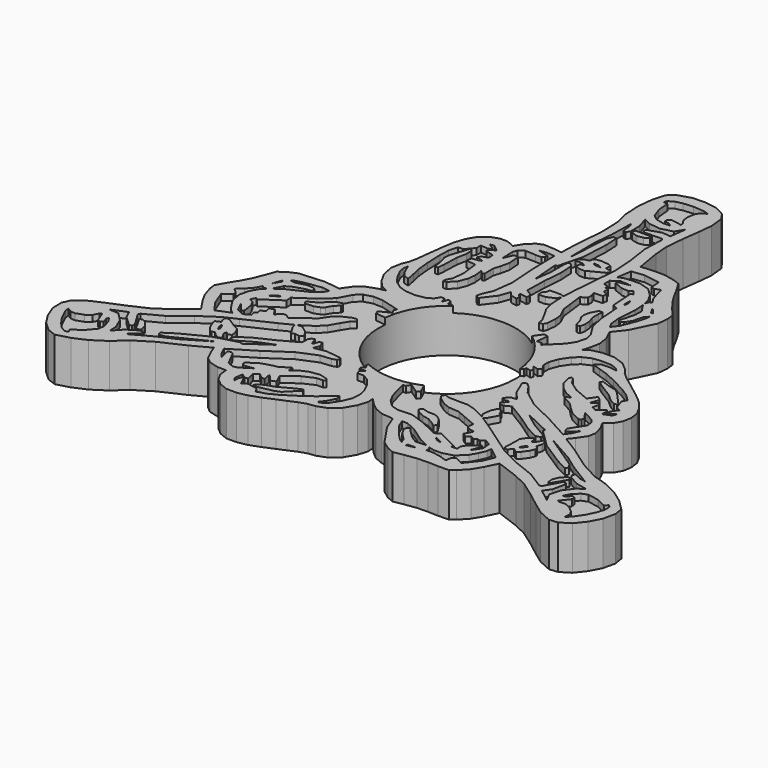
from build123d import *

# Parameters (mm, degrees)
F0_R            = 13.4
F0_R_2          = 11
F2_DEPTH        = 7
F3_DEPTH        = 7
F3_COPIES_COUNT = 3
F5_DEPTH        = 1
F5_COPIES_COUNT = 3
F6_R            = 0.2588079951
F6_R_2          = 0.2097461611
F6_R_3          = 0.2076285379
F7_DEPTH        = 7


# Not quite as in the source:
# - a pattern or mirror of a feature is missing from the dataset's text; its kind, count and spacing are read off the source's solid


with BuildPart() as f2:
    # F0 (on Top) → F2 (new body)
    with BuildSketch(Plane.XY):
        Circle(F0_R)
        Circle(F0_R_2, mode=Mode.SUBTRACT)
    extrude(amount=F2_DEPTH)

    # F1 (on Top) → F3 (join)
    with BuildSketch(Plane.XY):
        with BuildLine():
            ThreePointArc((-11.6641876562, 6.5959628805), (-0.1636582331, 13.3990005591), (11.4996029427, 6.8788903291))
            Line((11.4996029427, 6.8788903291), (12.5380335376, 7.9339332879))
            Line((12.5380335376, 7.9339332879), (13.6808827519, 9.3602091074))
            Line((13.6808827519, 9.3602091074), (14.2020219937, 11.0150557011))
            Line((14.2020219937, 11.0150557011), (14.4671630114, 12.5236166641))
            Line((14.4671630114, 12.5236166641), (14.256878756, 14.1144637018))
            Line((14.256878756, 14.1144637018), (13.4705984965, 15.7601684332))
            Line((13.4705984965, 15.7601684332), (14.9883022532, 17.6892988384))
            Line((14.9883022532, 17.6892988384), (16.7711470276, 21.3647019118))
            Line((16.7711470276, 21.3647019118), (16.9540029019, 23.0104047805))
            Line((16.9540029019, 23.0104047805), (16.8077182025, 24.2081098258))
            Line((16.8077182025, 24.2081098258), (15.7380122691, 25.497244671))
            Line((15.7380122691, 25.497244671), (14.6043049172, 26.941806078))
            Line((14.6043049172, 26.941806078), (13.6717399582, 28.4503661096))
            Line((13.6717399582, 28.4503661096), (12.9220308736, 29.8675000668))
            Line((12.9220308736, 29.8675000668), (12.0077515021, 31.3760600984))
            Line((12.0077515021, 31.3760600984), (11.1026149243, 31.741771847))
            Line((11.1026149243, 31.741771847), (9.3380557373, 32.1531966329))
            Line((9.3380557373, 32.1531966329), (7.6283533126, 32.1714803576))
            Line((7.6283533126, 32.1714803576), (5.4432251491, 32.0251956582))
            Line((5.4432251491, 32.0251956582), (4.7849440016, 35.9017364681))
            Line((4.7849440016, 35.9017364681), (4.6020881273, 38.2605791092))
            Line((4.6020881273, 38.2605791092), (4.8763719387, 41.2319898605))
            Line((4.8763719387, 41.2319898605), (5.2420832217, 44.0388247371))
            Line((5.2420832217, 44.0388247371), (5.4706535302, 46.2513826787))
            Line((5.4706535302, 46.2513826787), (5.242082756, 48.4639406204))
            Line((5.242082756, 48.4639406204), (4.4466597028, 49.5885051787))
            Line((4.4466597028, 49.5885051787), (2.8375282418, 50.4570677876))
            Line((2.8375282418, 50.4570677876), (0.8443988045, 50.7496409118))
            Line((0.8443988045, 50.7496409118), (-1.194444485, 50.6673529744))
            Line((-1.194444485, 50.6673529744), (-3.1052886043, 50.0639304519))
            Line((-3.1052886043, 50.0639304519), (-4.2572808452, 49.1222254932))
            Line((-4.2572808452, 49.1222254932), (-4.8241345212, 46.9736680388))
            Line((-4.8241345212, 46.9736680388), (-5.0709899515, 44.6788258851))
            Line((-5.0709899515, 44.6788258851), (-4.9338475801, 42.0639887452))
            Line((-4.9338475801, 42.0639887452), (-4.3761371635, 39.5588614047))
            Line((-4.3761371635, 39.5588614047), (-4.2755664326, 36.2948812544))
            Line((-4.2755664326, 36.2948812544), (-4.6504209749, 32.0617668331))
            Line((-4.6504209749, 32.0617668331), (-4.7601344995, 28.843505308))
            Line((-4.7601344995, 28.843505308), (-5.9669832699, 29.0355049074))
            Line((-5.9669832699, 29.0355049074), (-7.6675429009, 29.1452184319))
            Line((-7.6675429009, 29.1452184319), (-8.7372502312, 28.7429355085))
            Line((-8.7372502312, 28.7429355085), (-9.8709575832, 27.6092290878))
            Line((-9.8709575832, 27.6092290878), (-10.5749526992, 26.4389514923))
            Line((-10.5749526992, 26.4389514923), (-11.8823722005, 26.9875191152))
            Line((-11.8823722005, 26.9875191152), (-13.1257921457, 26.9875191152))
            Line((-13.1257921457, 26.9875191152), (-14.4240688533, 26.5212375671))
            Line((-14.4240688533, 26.5212375671), (-15.5669180676, 25.625243783))
            Line((-15.5669180676, 25.625243783), (-16.3989141583, 24.2081116885))
            Line((-16.3989141583, 24.2081116885), (-16.9291961938, 22.6721223444))
            Line((-16.9291961938, 22.6721223444), (-17.2400511801, 20.9167040884))
            Line((-17.2400511801, 20.9167040884), (-17.4686219543, 19.0150048584))
            Line((-17.4686219543, 19.0150048584), (-17.6514778286, 17.6253002137))
            Line((-17.6514778286, 17.6253002137), (-17.8069043905, 16.1898806691))
            Line((-17.8069043905, 16.1898806691), (-18.0811882019, 14.9098904803))
            Line((-18.0811882019, 14.9098904803), (-18.5291860253, 13.8401836157))
            Line((-18.5291860253, 13.8401836157), (-18.8020132482, 12.2613888234))
            Line((-18.8020132482, 12.2613888234), (-18.4454452246, 10.3779723868))
            Line((-18.4454452246, 10.3779723868), (-17.4945946783, 8.6956974119))
            Line((-17.4945946783, 8.6956974119), (-16.4157431573, 7.5345630758))
            Line((-16.4157431573, 7.5345630758), (-14.9711817503, 6.821425166))
            Line((-14.9711817503, 6.821425166), (-13.2554527372, 6.4937388524))
            Line((-13.2554527372, 6.4937388524), (-11.6641876562, 6.5959628805))
        make_face()
    f3 = extrude(amount=F3_DEPTH)

    # F3_copies: F3 ×3 about axis
    f3_copies_axis = Axis((0, 0, 0), (0, 0, 1))
    for i in range(1, F3_COPIES_COUNT):
        add(f3.rotate(f3_copies_axis, i * 360 / F3_COPIES_COUNT))

    # F4 (on face) → F5 (cut)
    with BuildSketch(Plane.XY.offset(7)):
        with BuildLine():
            Line((-6.7291953601, 9.3133719638), (-6.2807447637, 9.0306281738))
            ThreePointArc((-6.2807447637, 9.0306281738), (0.163569186, 10.9987838019), (6.5465070851, 8.8398667968))
            Line((6.5465070851, 8.8398667968), (7.4893734418, 10.1453736424))
            Line((7.4893734418, 10.1453736424), (8.0973692238, 10.0600402802))
            Line((8.0973692238, 10.0600402802), (7.9587036744, 8.1293871626))
            Line((7.9587036744, 8.1293871626), (8.7266983464, 8.1080542877))
            Line((8.7266983464, 8.1080542877), (8.9506972581, 7.692056708))
            Line((8.9506972581, 7.692056708), (11.1800152808, 9.9000418559))
            Line((11.1800152808, 9.9000418559), (11.9586763903, 11.1480327323))
            Line((11.9586763903, 11.1480327323), (12.3213399202, 12.5560229644))
            Line((12.3213399202, 12.5560229644), (12.0546752587, 13.7720145285))
            Line((12.0546752587, 13.7720145285), (10.8386827633, 15.6813338399))
            Line((10.8386827633, 15.6813338399), (10.3586865589, 18.0813185871))
            Line((10.3586865589, 18.0813185871), (10.1133547723, 21.3559605181))
            Line((10.1133547723, 21.3559605181), (9.2920269817, 21.7826254666))
            Line((9.2920269817, 21.7826254666), (9.0466951951, 25.4839323461))
            Line((9.0466951951, 25.4839323461), (9.4200260937, 25.601265952))
            Line((9.4200260937, 25.601265952), (8.8973622769, 26.3265930116))
            Line((8.8973622769, 26.3265930116), (8.3427000791, 25.9425956756))
            Line((8.3427000791, 25.9425956756), (7.2973738424, 25.9745959193))
            Line((7.2973738424, 25.9745959193), (5.6973844767, 26.6252588481))
            Line((5.6973844767, 26.6252588481), (5.8893831447, 26.9985888153))
            Line((5.8893831447, 26.9985888153), (7.7347038314, 27.2972546518))
            Line((7.7347038314, 27.2972546518), (5.8360504918, 27.414586395))
            Line((5.8360504918, 27.414586395), (4.7907242551, 26.646591723))
            Line((4.7907242551, 26.646591723), (4.7800578177, 25.5052670836))
            Line((4.7800578177, 25.5052670836), (5.4733860306, 25.3666006029))
            Line((5.4733860306, 25.3666006029), (5.5800522678, 24.8332712799))
            Line((5.5800522678, 24.8332712799), (6.0813818127, 24.6626045555))
            Line((6.0813818127, 24.6626045555), (6.0493825004, 23.8519441336))
            Line((6.0493825004, 23.8519441336), (6.7960438319, 23.6386116594))
            Line((6.7960438319, 23.6386116594), (6.7000444978, 22.8599514812))
            Line((6.7000444978, 22.8599514812), (5.2813878283, 22.774618119))
            Line((5.2813878283, 22.774618119), (5.5480524898, 22.0279563218))
            Line((5.5480524898, 22.0279563218), (5.5267191492, 21.3879607618))
            Line((5.5267191492, 21.3879607618), (5.1960549317, 21.0999622941))
            Line((5.1960549317, 21.0999622941), (4.6307253651, 20.8759643137))
            Line((4.6307253651, 20.8759643137), (4.9187233672, 18.5079798102))
            Line((4.9187233672, 18.5079798102), (5.0893891603, 17.0573238283))
            Line((5.0893891603, 17.0573238283), (5.8467173949, 15.4786678031))
            Line((5.8467173949, 15.4786678031), (5.9960498475, 14.3053419888))
            Line((5.9960498475, 14.3053419888), (5.8573838323, 12.7906855196))
            Line((5.8573838323, 12.7906855196), (5.5800522678, 12.2466897592))
            Line((5.5800522678, 12.2466897592), (4.9933898263, 12.1933566406))
            Line((4.9933898263, 12.1933566406), (4.8440573737, 13.0253508687))
            Line((4.8440573737, 13.0253508687), (4.2147282511, 14.2093431205))
            Line((4.2147282511, 14.2093431205), (3.3507344779, 15.7026667148))
            Line((3.3507344779, 15.7026667148), (2.9987369198, 17.0999895781))
            Line((2.9987369198, 17.0999895781), (2.8814044781, 19.3826407194))
            Line((2.8814044781, 19.3826407194), (2.550739795, 18.7426451594))
            Line((2.550739795, 18.7426451594), (1.228082343, 18.1773155928))
            Line((1.228082343, 18.1773155928), (0.1507562847, 18.1346479803))
            Line((0.1507562847, 18.1346479803), (0.022757129, 18.7639780343))
            Line((0.022757129, 18.7639780343), (0.4814206914, 19.339973107))
            Line((0.4814206914, 19.339973107), (0.5880866665, 19.8946371675))
            Line((0.5880866665, 19.8946371675), (2.4014078081, 19.9266355485))
            Line((2.4014078081, 19.9266355485), (2.9027375858, 19.7026375681))
            Line((2.9027375858, 19.7026375681), (3.0200700276, 21.8892898411))
            Line((3.0200700276, 21.8892898411), (3.4254004713, 26.8599223346))
            Line((3.4254004713, 26.8599223346), (3.6280651111, 29.2065739632))
            Line((3.6280651111, 29.2065739632), (3.3933999948, 32.5345508754))
            Line((3.3933999948, 32.5345508754), (2.8600706719, 36.1505262554))
            Line((2.8600706719, 36.1505262554), (2.9880695511, 39.3398366868))
            Line((2.9880695511, 39.3398366868), (2.7747380082, 39.6491698921))
            Line((2.7747380082, 39.6491698921), (-0.137241921, 39.5851694047))
            Line((-0.137241921, 39.5851694047), (-0.3612406144, 39.9158336222))
            Line((-0.3612406144, 39.9158336222), (-0.2652412222, 40.2784980834))
            Line((-0.2652412222, 40.2784980834), (1.8254109891, 40.9504920244))
            Line((1.8254109891, 40.9504920244), (3.1907348894, 40.8011600375))
            Line((3.1907348894, 40.8011600375), (3.5320662428, 43.4038117528))
            Line((3.5320662428, 43.4038117528), (2.7214051224, 42.1024858952))
            Line((2.7214051224, 42.1024858952), (0.8760846104, 41.6224896908))
            Line((0.8760846104, 41.6224896908), (-0.9799030377, 41.835822165))
            Line((-0.9799030377, 41.835822165), (-2.1425618324, 42.4331501126))
            Line((-2.1425618324, 42.4331501126), (-1.577232033, 40.6198278069))
            Line((-1.577232033, 40.6198278069), (-1.5345660504, 38.7745089829))
            Line((-1.5345660504, 38.7745089829), (-1.9078967161, 38.1878465414))
            Line((-1.9078967161, 38.1878465414), (-2.3665602785, 38.3265130222))
            Line((-2.3665602785, 38.3265130222), (-2.4732262827, 39.6385006607))
            Line((-2.4732262827, 39.6385006607), (-2.7505576145, 40.4064953327))
            Line((-2.7505576145, 40.4064953327), (-2.8572236188, 36.4278554916))
            Line((-2.8572236188, 36.4278554916), (-3.145221388, 33.5265398026))
            Line((-3.145221388, 33.5265398026), (-3.081221832, 28.523908928))
            Line((-3.081221832, 28.523908928), (-2.6438913774, 35.3505313396))
            Line((-2.6438913774, 35.3505313396), (-2.2385607008, 36.2038575113))
            Line((-2.2385607008, 36.2038575113), (-1.7265641363, 36.1611917615))
            Line((-1.7265641363, 36.1611917615), (-1.6198985977, 33.9212082326))
            Line((-1.6198985977, 33.9212082326), (-1.8332301406, 29.6119041741))
            Line((-1.8332301406, 29.6119041741), (-2.8358900454, 25.7079303265))
            Line((-2.8358900454, 25.7079303265), (-3.1772209331, 25.6439298391))
            Line((-3.1772209331, 25.6439298391), (-2.8145567048, 21.1319606751))
            Line((-2.8145567048, 21.1319606751), (-2.4412258063, 23.7559434026))
            Line((-2.4412258063, 23.7559434026), (-2.4305593688, 26.5719238669))
            Line((-2.4305593688, 26.5719238669), (-2.3132269271, 27.2119194269))
            Line((-2.3132269271, 27.2119194269), (-1.9718960393, 27.2439196706))
            Line((-1.9718960393, 27.2439196706), (-1.4598993585, 26.710588485))
            Line((-1.4598993585, 26.710588485), (-1.3319003629, 24.4706049562))
            Line((-1.3319003629, 24.4706049562), (-1.5772319166, 21.4946251363))
            Line((-1.5772319166, 21.4946251363), (-1.6518983757, 18.1559808552))
            Line((-1.6518983757, 18.1559808552), (-0.7239042316, 17.558651045))
            Line((-0.7239042316, 17.558651045), (-0.4785726778, 17.1213205904))
            Line((-0.4785726778, 17.1213205904), (-0.595905236, 16.6519898921))
            Line((-0.595905236, 16.6519898921), (-1.7798973713, 16.8759897351))
            Line((-1.7798973713, 16.8759897351), (-1.705231145, 16.545323655))
            Line((-1.705231145, 16.545323655), (-1.2359009124, 16.0759948194))
            Line((-1.2359009124, 16.0759948194), (-1.3425670331, 15.5853312463))
            Line((-1.3425670331, 15.5853312463), (-2.3452267051, 15.7773289829))
            Line((-2.3452267051, 15.7773289829), (-2.9425560497, 16.545323655))
            Line((-2.9425560497, 16.545323655), (-3.5612182692, 14.7853363305))
            Line((-3.5612182692, 14.7853363305), (-5.0865411758, 12.769350782))
            Line((-5.0865411758, 12.769350782), (-5.4385391995, 12.7586834133))
            Line((-5.4385391995, 12.7586834133), (-5.705203861, 13.0786811933))
            Line((-5.705203861, 13.0786811933), (-5.5345380679, 13.8466758654))
            Line((-5.5345380679, 13.8466758654), (-4.8305429518, 15.3933325782))
            Line((-4.8305429518, 15.3933325782), (-4.4252122752, 18.6146423221))
            Line((-4.4252122752, 18.6146423221), (-4.7345436178, 23.0092797428))
            Line((-4.7345436178, 23.0092797428), (-4.8412093893, 27.5532491505))
            Line((-4.8412093893, 27.5532491505), (-6.0038683005, 27.6599153876))
            Line((-6.0038683005, 27.6599153876), (-7.2198598646, 27.5319162756))
            Line((-7.2198598646, 27.5319162756), (-5.5238711648, 27.0412527025))
            Line((-5.5238711648, 27.0412527025), (-5.5558704771, 26.5612564981))
            Line((-5.5558704771, 26.5612564981), (-5.8972020634, 26.2839253992))
            Line((-5.8972020634, 26.2839253992), (-6.8678618409, 26.3159237802))
            Line((-6.8678618409, 26.3159237802), (-8.563850075, 26.4012571424))
            Line((-8.563850075, 26.4012571424), (-9.3638449907, 25.8145947009))
            Line((-9.3638449907, 25.8145947009), (-9.6198432148, 25.1319315284))
            Line((-9.6198432148, 25.1319315284), (-9.5451772213, 23.0199471116))
            Line((-9.5451772213, 23.0199471116), (-8.9265145361, 24.5132707059))
            Line((-8.9265145361, 24.5132707059), (-8.4678512067, 24.6199350804))
            Line((-8.4678512067, 24.6199350804), (-8.1691863015, 24.4066044688))
            Line((-8.1691863015, 24.4066044688), (-8.0411871895, 22.5719492882))
            Line((-8.0411871895, 22.5719492882), (-8.3611849695, 21.1212933064))
            Line((-8.3611849695, 21.1212933064), (-8.6811827496, 20.1399661601))
            Line((-8.6811827496, 20.1399661601), (-8.6598489434, 18.3479785919))
            Line((-8.6598489434, 18.3479785919), (-8.9585138485, 18.2093121111))
            Line((-8.9585138485, 18.2093121111), (-9.4598438591, 18.6999756843))
            Line((-9.4598438591, 18.6999756843), (-9.2998445034, 17.20665209))
            Line((-9.2998445034, 17.20665209), (-9.4385109842, 16.0226598382))
            Line((-9.4385109842, 16.0226598382), (-10.0038396195, 14.5720038563))
            Line((-10.0038396195, 14.5720038563), (-10.9745003283, 13.6226769537))
            Line((-10.9745003283, 13.6226769537), (-11.4651629701, 13.5480109602))
            Line((-11.4651629701, 13.5480109602), (-11.4758303389, 13.9640085399))
            Line((-11.4758303389, 13.9640085399), (-10.9638338909, 14.9026690051))
            Line((-10.9638338909, 14.9026690051), (-10.7825016603, 16.9079881161))
            Line((-10.7825016603, 16.9079881161), (-11.1238332465, 19.5426363498))
            Line((-11.1238332465, 19.5426363498), (-12.6598225906, 19.7026357055))
            Line((-12.6598225906, 19.7026357055), (-12.5104906037, 20.5346290022))
            Line((-12.5104906037, 20.5346290022), (-11.3691650331, 20.7159612328))
            Line((-11.3691650331, 20.7159612328), (-11.0278343782, 20.8759605885))
            Line((-11.0278343782, 20.8759605885), (-12.1798263863, 21.2706252933))
            Line((-12.1798263863, 21.2706252933), (-11.9238281623, 21.7292886227))
            Line((-11.9238281623, 21.7292886227), (-10.9318345785, 22.0492854714))
            Line((-10.9318345785, 22.0492854714), (-11.0278343782, 22.9239463806))
            Line((-11.0278343782, 22.9239463806), (-11.6891628131, 23.1052786112))
            Line((-11.6891628131, 23.1052786112), (-12.3718250543, 23.3399439603))
            Line((-12.3718250543, 23.3399439603), (-12.1691590175, 23.8412730396))
            Line((-12.1691590175, 23.8412730396), (-11.3798314705, 24.1826046258))
            Line((-11.3798314705, 24.1826046258), (-12.4678239226, 25.057265535))
            Line((-12.4678239226, 25.057265535), (-13.1291532889, 24.929266423))
            Line((-13.1291532889, 24.929266423), (-12.4144908041, 24.5239362121))
            Line((-12.4144908041, 24.5239362121), (-12.2224921361, 24.0972712636))
            Line((-12.2224921361, 24.0972712636), (-12.5851565972, 23.9159408957))
            Line((-12.5851565972, 23.9159408957), (-13.7904807925, 24.0119379014))
            Line((-13.7904807925, 24.0119379014), (-13.8118136674, 23.1372769922))
            Line((-13.8118136674, 23.1372769922), (-14.9104734883, 21.878618747))
            Line((-14.9104734883, 21.878618747), (-15.7424677163, 21.878618747))
            Line((-15.7424677163, 21.878618747), (-16.1051321775, 20.44929564))
            Line((-16.1051321775, 20.44929564), (-16.190463677, 18.79597269))
            Line((-16.190463677, 18.79597269), (-16.0731300712, 16.1186587065))
            Line((-16.0731300712, 16.1186587065), (-15.8704649657, 14.1026722267))
            Line((-15.8704649657, 14.1026722267), (-15.550468117, 12.6840155572))
            Line((-15.550468117, 12.6840155572), (-15.2944689617, 11.3080246374))
            Line((-15.2944689617, 11.3080246374), (-16.1371305585, 11.553356424))
            Line((-16.1371305585, 11.553356424), (-16.8411247432, 12.5773493201))
            Line((-16.8411247432, 12.5773493201), (-17.3744559288, 13.8680078089))
            Line((-17.3744559288, 13.8680078089), (-17.5237879157, 13.1960120052))
            Line((-17.5237879157, 13.1960120052), (-17.36378856, 12.25735154))
            Line((-17.36378856, 12.25735154), (-16.6064612567, 10.7746953145))
            Line((-16.6064612567, 10.7746953145), (-15.7744660974, 9.6653699875))
            Line((-15.7744660974, 9.6653699875), (-14.6011412144, 8.8440421969))
            Line((-14.6011412144, 8.8440421969), (-13.4171498939, 8.4600448608))
            Line((-13.4171498939, 8.4600448608), (-11.806493625, 8.3533786237))
            Line((-11.806493625, 8.3533786237), (-10.3665040806, 8.5987104103))
            Line((-10.3665040806, 8.5987104103), (-9.3958433717, 9.1320406646))
            Line((-9.3958433717, 9.1320406646), (-8.9265136048, 9.9853677675))
            Line((-8.9265136048, 9.9853677675), (-8.3185173571, 9.9213682115))
            Line((-8.3185173571, 9.9213682115), (-8.1265186891, 8.9933741838))
            Line((-8.1265186891, 8.9933741838), (-7.7425218187, 9.932034649))
            Line((-7.7425218187, 9.932034649), (-7.3051913641, 9.8573686555))
            Line((-7.3051913641, 9.8573686555), (-7.1131926961, 9.078707546))
            Line((-7.1131926961, 9.078707546), (-6.7291953601, 9.3133719638))
        make_face()
        Polygon((-14.2694124952, 16.0346571356), (-14.7294998169, 16.0120297223), (-14.9859422818, 17.399834469), (-15.34043625, 18.6745040119), (-15.2046727017, 19.6248479187), (-14.5861944184, 21.5179957449), (-14.2920399085, 22.4155448377), (-14.1034796834, 22.4607996643), (-13.8168670237, 22.128932178), (-13.7866977602, 21.0956204683), (-14.0883941203, 19.5871386677), (-14.1638182104, 17.0453414321), align=None, mode=Mode.SUBTRACT)
        Polygon((9.1748032719, 14.6242082119), (8.9334454387, 14.790141955), (8.7222578004, 15.7329440117), (8.1867454574, 16.6531186551), (8.0811521038, 17.3017680645), (8.2244575024, 18.1917734444), (8.8655631989, 19.3985607475), (9.4312448055, 19.3910188973), (9.3407360837, 18.6820309609), (9.3407360837, 17.5355821848), (9.6876872703, 16.4645593613), (9.7706541419, 15.4387895018), (9.5971785486, 14.6694630384), align=None, mode=Mode.SUBTRACT)
        Polygon((-1.4074409846, 29.1237011552), (-0.5575600662, 29.33299914), (-0.4687665205, 29.8150219023), (-0.1453044388, 30.0687178969), (0.6411524955, 30.1575101912), (1.801810693, 30.0623755902), (2.3916533682, 29.8086795956), (2.3028599098, 28.9841685444), (3.1400558073, 28.8192648441), (3.4000941087, 28.527515009), (3.1527406536, 28.0835479498), (1.2309951708, 27.0941331983), (0.7109188009, 26.7516449094), (-0.2975219395, 26.80872567), (-0.9888429195, 27.1512158215), (-0.9190765559, 27.7727711946), (-0.3609458217, 27.8932750225), (-0.7605166757, 28.2167382538), (-1.9845988136, 28.2294228673), (-1.9275173545, 28.7431571633), align=None, mode=Mode.SUBTRACT)
        Polygon((-1.2926241616, 38.7684516609), (-1.144627342, 39.2886847258), (1.4777268559, 39.2639720491), (1.5103446785, 38.8626307249), (0.8062389097, 38.405187428), (-0.1355586282, 38.2796153426), (-1.1760205962, 38.5487005115), align=None, mode=Mode.SUBTRACT)
        Polygon((5.2816621028, 30.2993506193), (4.9497955479, 27.9612001032), (5.6663253345, 28.2855238765), (6.8806554191, 28.4062027931), (8.1854937598, 28.4439157695), (9.9504208192, 27.9084034264), (11.1647499725, 26.7317853868), (11.8284830824, 25.5777947605), (12.0849255472, 24.6349927038), (12.3111987486, 25.1931324601), (12.6883191988, 25.2987258136), (12.100010179, 26.2716971338), (11.7002623156, 27.4784844369), (11.4287352189, 28.7380684167), (10.5161024258, 28.4062027931), (9.965505451, 28.6023057997), (9.8523693159, 30.1560442895), (7.287946064, 30.5482503027), align=None)
        Polygon((13.0964461714, 22.670423612), (12.1705643833, 24.0998845547), (12.2916530818, 22.3822239786), (12.1974730864, 21.2475825101), (12.0405070484, 19.3819273263), (12.2215254232, 17.6622569561), (12.6439006999, 16.8325901031), (13.4433973581, 17.8885292262), (14.348488301, 20.1512556523), (14.7256096825, 21.4636363089), (14.7708635777, 22.1273694187), (14.2428940162, 21.5088911355), (13.8356033713, 19.9551526457), (13.2322097197, 18.9595520496), (12.7645805478, 18.763449043), (12.3422043398, 19.0198924392), (12.6891555265, 19.8948122561), (13.0813615397, 21.5692296624), align=None)
        Polygon((10.2138053626, 24.1370685399), (10.2326609194, 22.7341782302), (10.3835100308, 22.7002371103), (10.440078564, 23.3111735433), align=None)
        Polygon((14.5914833993, 23.0984371156), (13.5834896937, 24.2610964924), (14.2768183723, 23.0557713658), align=None)
        Polygon((1.1552217184, 29.0367566049), (0.2941497078, 29.0905740112), (0.6170517299, 28.790095821), (1.6306053149, 28.7497323006), align=None)
        Polygon((-3.0859704129, 48.0316206813), (-3.2381881028, 47.5242286921), (-2.603948582, 47.4354363978), (-2.4580736645, 45.6405393779), (-1.8618884496, 43.9598038793), (-1.0817738948, 43.3382466435), (0.2881833643, 42.9957583547), (1.3156513451, 43.0655255914), (0.9668194689, 43.3763042092), (0.135965849, 43.5919426382), (0.0788842663, 44.0168827772), (0.4974823678, 44.3403460085), (2.286037663, 44.0676249564), (2.286037663, 44.4164536893), (1.75961887, 45.2029109001), (1.6327708727, 46.2494082749), (1.8674397143, 47.4544614553), (2.2733530495, 48.0823591352), (3.0661521014, 48.4882704914), (2.2987225093, 48.7546510994), (0.3896617563, 48.9068701863), (-1.1261705076, 48.7800240517), (-2.2424319759, 48.5263280571), align=None)
    f5 = extrude(amount=-F5_DEPTH, mode=Mode.SUBTRACT)

    # F5_copies: F5 ×3 about axis
    f5_copies_axis = Axis((0, 0, 0), (0, 0, 1))
    for i in range(1, F5_COPIES_COUNT):
        add(f5.rotate(f5_copies_axis, i * 360 / F5_COPIES_COUNT), mode=Mode.SUBTRACT)

    # F6 (on face) → F7 (join)
    with BuildSketch(Plane.XY.offset(7)):
        with Locations((0.1724938629, -13.4378448129)):
            Circle(F6_R)
        with Locations((-11.7595139891, 6.5683354624)):
            Circle(F6_R_2)
        with Locations((11.5623343736, 6.914707832)):
            Circle(F6_R_3)
    extrude(amount=-F7_DEPTH)


solid = f2.part
